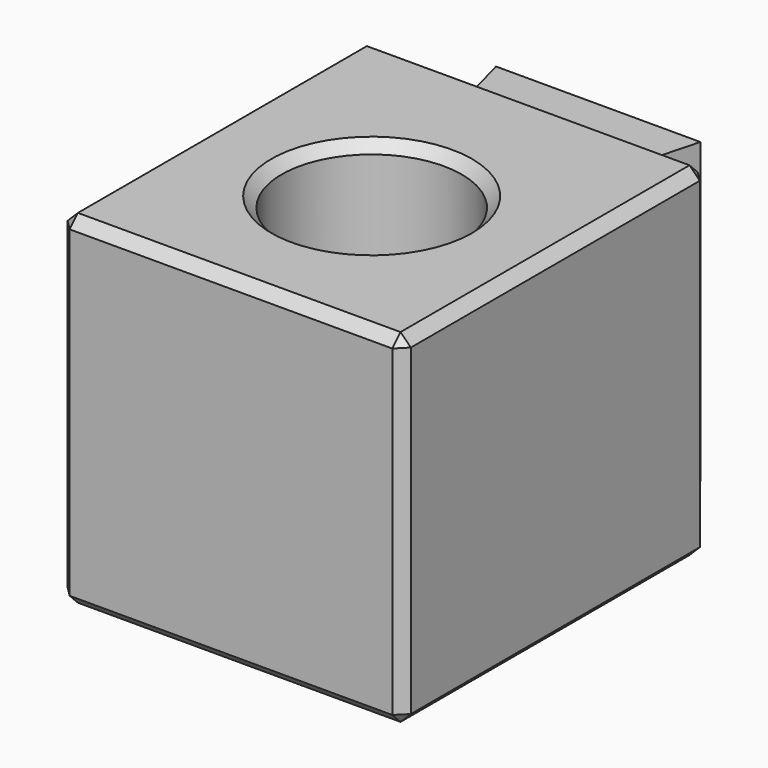
from build123d import *

# Parameters (mm, degrees)
F2_R     = 5.25
F3_DEPTH = 20
F4_DEPTH = 18
F5_SIZE  = 0.6


# Not quite as in the source:
# - a feature names something its author has since deleted; it is built from what else it names


with BuildPart() as f3:
    # F2 (on Top) → F3 (new body)
    with BuildSketch(Plane.XY):
        Polygon((5.25, 22.25), (0, 22.25), (0, 0), (20, 0), (20, 22.25), (14.75, 22.25), align=None)
        with Locations((10, 10.25)):
            Circle(F2_R, mode=Mode.SUBTRACT)
    extrude(amount=F3_DEPTH)

    # F2 (on Top) → F4 (join)
    with BuildSketch(Plane.XY):
        Polygon((4.0442286341, 26.75), (5.25, 22.25), (14.75, 22.25), (15.9557713659, 26.75), align=None)
    extrude(amount=F4_DEPTH)

    # F5
    f5_edges = [f3.edges().sort_by_distance(p)[0] for p in [
        (0, 11.125, 0),
        (10, 0, 0),
        (20, 11.125, 0),
        (17.375, 22.25, 0),
        (15.352886, 24.5, 0),
        (10, 26.75, 0),
        (4.647114, 24.5, 0),
        (2.625, 22.25, 0),
        (4.75, 10.25, 0),
        (10, 22.25, 20),
        (0, 11.125, 20),
        (10, 0, 20),
        (20, 11.125, 20),
        (4.75, 10.25, 20),
        (0, 0, 10),
        (20, 0, 10),
        (20, 22.25, 10),
    ]]
    chamfer(f5_edges, length=F5_SIZE)


solid = f3.part
